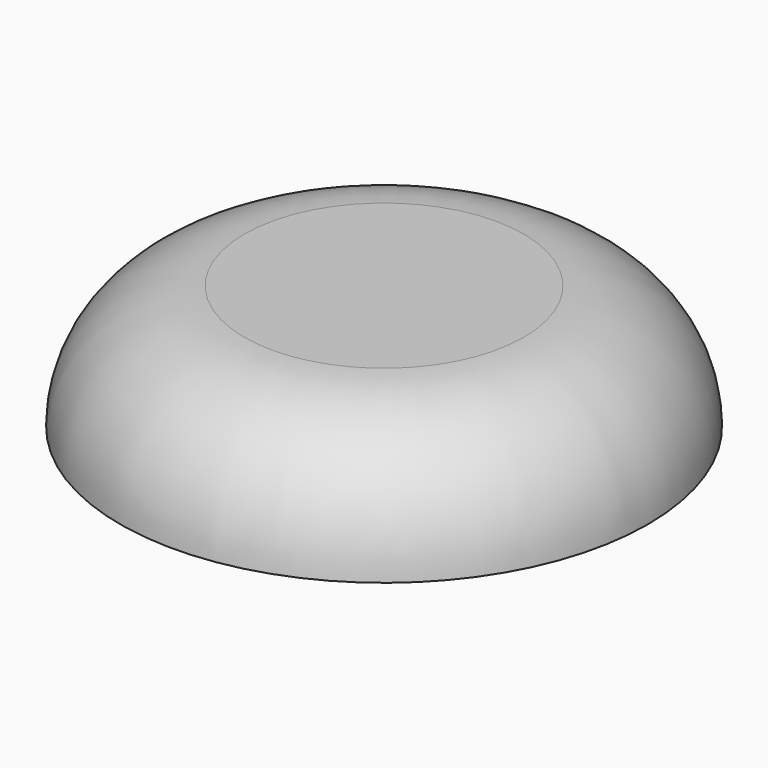
from build123d import *

# Parameters (mm, degrees)
F0_R     = 4.25
F1_DEPTH = 2
F2_R     = 1.99999


# Not quite as in the source:
# - a fillet or chamfer is up to 0.001 mm smaller than in the source, because OpenCascade refuses the exact size


with BuildPart() as f1:
    # F0 (on Top) → F1 (new body)
    with BuildSketch(Plane.XY):
        Circle(F0_R)
    extrude(amount=F1_DEPTH)

    # F2 (radius 2 in the source; OpenCascade refuses exactly that, so slightly less here)
    f2_edges = [f1.edges().sort_by_distance(p)[0] for p in [
        (-4.25, 0, 2),
    ]]
    fillet(f2_edges, radius=F2_R)


solid = f1.part
